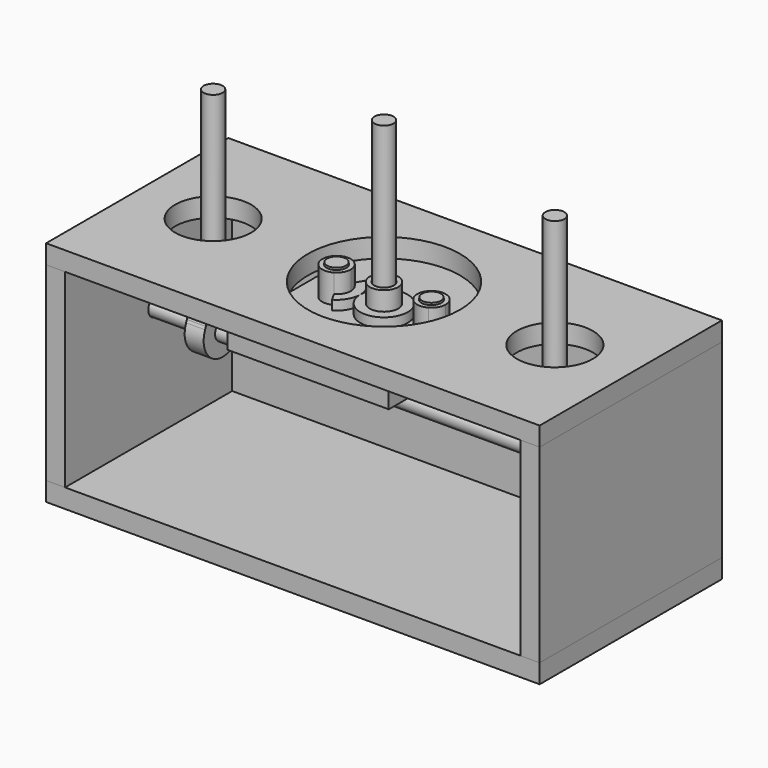
from build123d import *
from build123d import SkipClean  # not in build123d's __all__

# Parameters (mm, degrees)
F0_W           = 304.8
F0_H           = 12.7
F0_H_2         = 127
F1_DEPTH       = 12.7
F2_DEPTH       = 127
F3_DEPTH       = 127
F4_DEPTH       = 127
F5_START       = -139.7
F1_FACE_W      = 330.2
F1_FACE_H      = 152.4
F5_DEPTH       = 12.7
F6_R           = 25.4
F6_R_2         = 50.8
F7_DEPTH       = 12.7
F8_R           = 6.604
F8_R_2         = 6.35
F9_DEPTH       = 12.7
F10_R          = 6.604
F11_DEPTH      = 6.35
F12_DEPTH      = 323.85
F12_DEPTH_BACK = 25.4
F14_START      = 31.75
F13_R          = 6.35
F14_DEPTH      = 12.7
F15_R          = 6.604
F16_DEPTH      = 6.35
F15_R_2        = 9.525
F17_DEPTH      = 12.7
F18_W          = 107.95
F18_H          = 12.7
F19_DEPTH      = 127
F20_R          = 6.604
F21_DEPTH      = 12.7
F22_R          = 6.35
F23_DEPTH      = 12.7
F23_DEPTH_BACK = 33.02
F24_DEPTH      = 6.35
F24_DEPTH_BACK = 127
F25_R          = 6.35
F26_DEPTH      = 76.2
F26_DEPTH_BACK = 35.56


# Not quite as in the source:
# - a pattern or mirror of a feature is missing from the dataset's text; its kind, count and spacing are read off the source's solid


with BuildPart() as f1:
    # F0 (on Top) → F1 (new body)
    with BuildSketch(Plane.XY):
        with Locations((0, 69.85)):
            Rectangle(F0_W, F0_H)
        Polygon((-152.4, 76.2), (-165.1, 76.2), (-165.1, -76.2), (-152.4, -76.2), (-152.4, -63.5), (-152.4, 63.5), align=None)
        Rectangle(F0_W, F0_H_2)
        with Locations((0, -69.85)):
            Rectangle(F0_W, F0_H)
        Polygon((165.1, 76.2), (152.4, 76.2), (152.4, 63.5), (152.4, -63.5), (152.4, -76.2), (165.1, -76.2), align=None)
    extrude(amount=-F1_DEPTH)


with BuildPart() as f2:
    # F0 (on Top) → F2 (new body)
    with BuildSketch(Plane.XY):
        with Locations((0, 69.85)):
            Rectangle(F0_W, F0_H)
    extrude(amount=F2_DEPTH)


with BuildPart() as f3:
    # F0 (on Top) → F3 (new body)
    with BuildSketch(Plane.XY):
        Polygon((-152.4, 76.2), (-165.1, 76.2), (-165.1, -76.2), (-152.4, -76.2), (-152.4, -63.5), (-152.4, 63.5), align=None)
    extrude(amount=F3_DEPTH)

    # F8 (on face) → F9 (cut)
    with BuildSketch(Plane(origin=(-165.1, 0, 0), x_dir=(0, -1, 0), z_dir=(-1, 0, 0))):
        with Locations((0, 76.2)):
            Circle(F8_R)
        with Locations((0, 76.2)):
            Circle(F8_R_2, mode=Mode.SUBTRACT)
    extrude(amount=-F9_DEPTH, mode=Mode.SUBTRACT)


with BuildPart() as f4:
    # F0 (on Top) → F4 (new body)
    with BuildSketch(Plane.XY):
        Polygon((165.1, 76.2), (152.4, 76.2), (152.4, 63.5), (152.4, -63.5), (152.4, -76.2), (165.1, -76.2), align=None)
    extrude(amount=F4_DEPTH)

    # F10 (on face) → F11 (cut)
    with BuildSketch(Plane(origin=(152.4, 0, 0), x_dir=(0, -1, 0), z_dir=(-1, 0, 0))):
        with Locations((0, 76.2)):
            Circle(F10_R)
    extrude(amount=-F11_DEPTH, mode=Mode.SUBTRACT)


with BuildPart() as f5:
    # F1_face (on face) → F5 (new body)
    with BuildSketch(Plane(origin=(0, 0, -12.7), x_dir=(1, 0, 0), z_dir=(0, 0, -1)).offset(F5_START)):
        Rectangle(F1_FACE_W, F1_FACE_H)
    extrude(amount=-F5_DEPTH)

    # F6 (on face) → F7 (cut)
    with BuildSketch(Plane.XY.offset(139.7)):
        with Locations((-114.3, 0)):
            Circle(F6_R)
        Circle(F6_R_2)
        with Locations((114.3, 0)):
            Circle(F6_R)
    extrude(amount=-F7_DEPTH, mode=Mode.SUBTRACT)


with BuildPart() as f12:
    # F12 (new, two sides): a face of the model
    f12_faces = [f3.part.faces().sort_by_distance(p)[0] for p in [
        (-165.1, 0, 76.2),
    ]]
    extrude(f12_faces, amount=-F12_DEPTH)
    extrude(f12_faces, amount=F12_DEPTH_BACK)


with BuildPart() as f14:
    # F13 (on face) → F14 (new body)
    with BuildSketch(Plane.YZ.offset(-152.4).offset(F14_START)):
        with BuildLine():
            ThreePointArc((-14.0285273832, 83.9985161394), (-14.335237854, 83.122228751), (-14.67376788, 82.25773565))
            ThreePointArc((-14.67376788, 82.25773565), (0, 60.325), (14.67376788, 82.25773565))
            ThreePointArc((14.67376788, 82.25773565), (14.335237854, 83.122228751), (14.0285273832, 83.9985161394))
            Line((14.0285273832, 83.9985161394), (10.2523893695, 95.454428534))
            ThreePointArc((10.2523893695, 95.454428534), (0, 102.87), (-10.2523893695, 95.454428534))
            Line((-10.2523893695, 95.454428534), (-14.0285273832, 83.9985161394))
        make_face()
        with Locations((0, 76.2)):
            Circle(F13_R, mode=Mode.SUBTRACT)
    extrude(amount=F14_DEPTH)


with BuildPart() as f14_copies_1:
    # F14_copies: instance of F14
    add(f14.part.mirror(Plane(origin=(0, 0, 0), x_dir=(0, 0, 1), z_dir=(1, 0, 0))), clean=False)


with BuildPart() as f16:
    # F15 (on face) → F16 (new body)
    with BuildSketch(Plane(origin=(0, 0, 127), x_dir=(1, 0, 0), z_dir=(0, 0, -1))):
        with BuildLine():
            ThreePointArc((-26.9875, 8.248891971), (-41.275, 0), (-26.9875, -8.248891971))
            ThreePointArc((-26.9875, -8.248891971), (-23.501108029, -4.7625), (-22.225, 0))
            ThreePointArc((-22.225, 0), (-23.501108029, 4.7625), (-26.9875, 8.248891971))
        make_face()
        with Locations((-31.75, 0)):
            Circle(F15_R, mode=Mode.SUBTRACT)
        with BuildLine():
            ThreePointArc((-23.8125, -13.7481532851), (-18.0018467087, -7.9374999892), (-15.875, 2.48e-08))
            ThreePointArc((-15.875, 2.48e-08), (-18.0018467211, 7.9375000108), (-23.8125, 13.7481532851))
            Line((-23.8125, 13.7481532851), (-26.9875, 8.248891971))
            ThreePointArc((-26.9875, 8.248891971), (-23.501108029, 4.7625), (-22.225, 0))
            ThreePointArc((-22.225, 0), (-23.501108029, -4.7625), (-26.9875, -8.248891971))
            Line((-26.9875, -8.248891971), (-23.8125, -13.7481532851))
        make_face()
    extrude(amount=F16_DEPTH)

    # F15 (on face) → F17 (join)
    with BuildSketch(Plane(origin=(0, 0, 127), x_dir=(1, 0, 0), z_dir=(0, 0, -1))):
        with BuildLine():
            ThreePointArc((-26.9875, 8.248891971), (-41.275, 0), (-26.9875, -8.248891971))
            ThreePointArc((-26.9875, -8.248891971), (-23.501108029, -4.7625), (-22.225, 0))
            ThreePointArc((-22.225, 0), (-23.501108029, 4.7625), (-26.9875, 8.248891971))
        make_face()
        with Locations((-31.75, 0)):
            Circle(F15_R, mode=Mode.SUBTRACT)
    extrude(amount=-F17_DEPTH)


with BuildPart() as f16b:
    # F15 (on face) → F16, piece 2 (new body)
    with BuildSketch(Plane(origin=(0, 0, 127), x_dir=(1, 0, 0), z_dir=(0, 0, -1))):
        with BuildLine():
            ThreePointArc((-15.875, 2.48e-08), (-1.24e-08, -15.875), (15.875, 0))
            ThreePointArc((15.875, 0), (1.24e-08, 15.875), (-15.875, 2.48e-08))
        make_face()
        Circle(F15_R_2, mode=Mode.SUBTRACT)
        Circle(F15_R_2)
        Circle(F15_R, mode=Mode.SUBTRACT)
    extrude(amount=F16_DEPTH)

    # F15 (on face) → F17, piece 2 (join)
    with BuildSketch(Plane(origin=(0, 0, 127), x_dir=(1, 0, 0), z_dir=(0, 0, -1))):
        Circle(F15_R_2)
        Circle(F15_R, mode=Mode.SUBTRACT)
    extrude(amount=-F17_DEPTH)


with BuildPart() as f16c:
    # F15 (on face) → F16, piece 3 (new body)
    with BuildSketch(Plane(origin=(0, 0, 127), x_dir=(1, 0, 0), z_dir=(0, 0, -1))):
        with BuildLine():
            ThreePointArc((36.5125, -8.248891971), (39.998891971, -4.7625), (41.275, 0))
            ThreePointArc((41.275, 0), (39.998891971, 4.7625), (36.5125, 8.248891971))
            ThreePointArc((36.5125, 8.248891971), (22.225, 0), (36.5125, -8.248891971))
        make_face()
        with Locations((31.75, 0)):
            Circle(F15_R, mode=Mode.SUBTRACT)
        with BuildLine():
            ThreePointArc((36.5125, 8.248891971), (39.998891971, 4.7625), (41.275, 0))
            ThreePointArc((41.275, 0), (39.998891971, -4.7625), (36.5125, -8.248891971))
            Line((36.5125, -8.248891971), (39.6875, -13.7481532851))
            ThreePointArc((39.6875, -13.7481532851), (47.625, 0), (39.6875, 13.7481532851))
            Line((39.6875, 13.7481532851), (36.5125, 8.248891971))
        make_face()
    extrude(amount=F16_DEPTH)

    # F15 (on face) → F17, piece 3 (join)
    with BuildSketch(Plane(origin=(0, 0, 127), x_dir=(1, 0, 0), z_dir=(0, 0, -1))):
        with BuildLine():
            ThreePointArc((36.5125, -8.248891971), (39.998891971, -4.7625), (41.275, 0))
            ThreePointArc((41.275, 0), (39.998891971, 4.7625), (36.5125, 8.248891971))
            ThreePointArc((36.5125, 8.248891971), (22.225, 0), (36.5125, -8.248891971))
        make_face()
        with Locations((31.75, 0)):
            Circle(F15_R, mode=Mode.SUBTRACT)
    with SkipClean():  # cleaning this boolean's faces spoils the solid; the shape is the same uncleaned
        extrude(amount=-F17_DEPTH)


with BuildPart() as f19:
    # F18 (on face) → F19 (new body)
    with BuildSketch(Plane.XZ.offset(-63.5)):
        with Locations((0, 114.3)):
            Rectangle(F18_W, F18_H)
    extrude(amount=F19_DEPTH)

    # F20 (on face) → F21 (cut)
    with BuildSketch(Plane(origin=(0, 0, 107.95), x_dir=(1, 0, 0), z_dir=(0, 0, -1))):
        with Locations((-31.75, 0)):
            Circle(F20_R)
        Circle(F20_R)
        with Locations((31.75, 0)):
            Circle(F20_R)
    extrude(amount=-F21_DEPTH, mode=Mode.SUBTRACT)


with BuildPart() as f23:
    # F22 (on face) → F23 (new body, two sides)
    with BuildSketch(Plane(origin=(0, 0, 107.95), x_dir=(1, 0, 0), z_dir=(0, 0, -1))) as f23_sk:
        with Locations((-31.75, 0)):
            Circle(F22_R)
    extrude(amount=F23_DEPTH)
    extrude(f23_sk.sketch, amount=-F23_DEPTH_BACK)


with BuildPart() as f23b:
    # F22 (on face) → F23, piece 2 (new body, two sides)
    with BuildSketch(Plane(origin=(0, 0, 107.95), x_dir=(1, 0, 0), z_dir=(0, 0, -1))) as f23_2_sk:
        with Locations((31.75, 0)):
            Circle(F22_R)
    extrude(amount=F23_DEPTH)
    extrude(f23_2_sk.sketch, amount=-F23_DEPTH_BACK)


with BuildPart() as f24:
    # F22 (on face) → F24 (new body, two sides)
    with BuildSketch(Plane(origin=(0, 0, 107.95), x_dir=(1, 0, 0), z_dir=(0, 0, -1))) as f24_sk:
        Circle(F22_R)
    extrude(amount=F24_DEPTH)
    extrude(f24_sk.sketch, amount=-F24_DEPTH_BACK)


with BuildPart() as f26:
    # F25 (on face) → F26 (new body, two sides)
    with BuildSketch(Plane.XY.offset(139.7)) as f26_sk:
        with Locations((-114.3, 0)):
            Circle(F25_R)
    extrude(amount=F26_DEPTH)
    extrude(f26_sk.sketch, amount=-F26_DEPTH_BACK)


with BuildPart() as f27_1:
    # F27: instance of F26
    add(f26.part.mirror(Plane.YZ), clean=False)


solid = Compound([f1.part, f2.part, f3.part, f4.part, f5.part, f12.part, f14.part, f14_copies_1.part, f16.part, f16b.part, f16c.part, f19.part, f23.part, f23b.part, f24.part, f26.part, f27_1.part])
